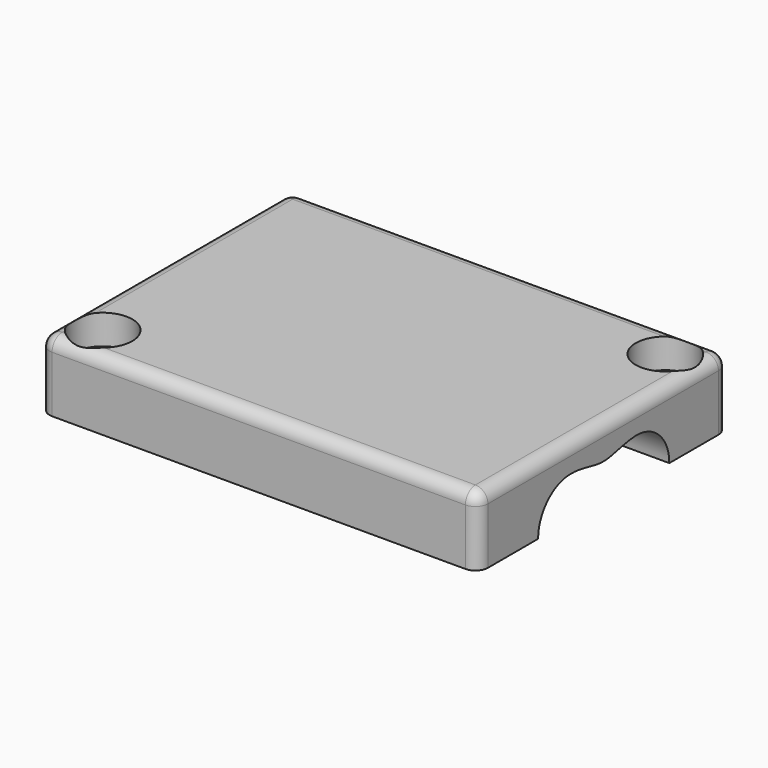
from build123d import *

# Parameters (mm, degrees)
F1_W          = 44.45
F1_H          = 31.75
F2_DEPTH      = 6.985
F4_DEPTH      = 44.45
F6_W          = 31.875
F6_H          = 1.75
F6_W_2        = 31.877
F7_DEPTH      = 2.5
F7_TAPER      = 7
F5_R          = 1.6
F8_DEPTH      = 25.4
F9_R          = 3
F9_R_2        = 1.6
F10_DEPTH     = 3
F11_T1_DEPTH  = 29.21
F11_T3_DEPTH  = 8.89
F11_T5_DEPTH  = 41.91
F11_S9_W      = 1.27
F11_S9_H      = 1.27
F11_T10_DEPTH = 1.27
F11_S15_W     = 1.27
F11_S15_H     = 1.27
F11_T16_DEPTH = 1.27
F11_S21_W     = 1.27
F11_S21_H     = 1.27
F11_T22_DEPTH = 1.27
F11_S27_W     = 1.27
F11_S27_H     = 1.27
F11_T28_DEPTH = 1.27


# Not quite as in the source:
# - a fillet or chamfer that OpenCascade refuses, or shapes differently, is made with other operations: its cross-section is extruded or revolved along the edge and cut away or added


with BuildPart() as f2:
    # F1 (on Top) → F2 (new body)
    with BuildSketch(Plane.XY):
        Rectangle(F1_W, F1_H)
    extrude(amount=F2_DEPTH)

    # F3 (on face) → F4 (cut, through all)
    with BuildSketch(Plane.YZ.offset(22.225)):
        with BuildLine():
            add(Edge.make_bspline(
                [(-4.125, 4.125), (-2.4255892558, 4.1137489608), (-0.0276085061, 2.971292738), (2.5249406681, 4.1137612248), (4.191, 4.191)],
                knots=[0, 0, 0, 0, 0.4977710734, 1, 1, 1, 1], degree=3))
            ThreePointArc((-4.125, 4.125), (-7.0418154724, 2.9168154724), (-8.25, 0))
            ThreePointArc((-8.25, 0), (-7.0418154724, -2.9168154724), (-4.125, -4.125))
            add(Edge.make_bspline(
                [(-4.125, -4.125), (-2.9335741419, -4.2006121948), (0.4172014685, -3.0581585459), (2.1438994445, -4.2006121948), (4.191, -4.191)],
                knots=[0, 0, 0, 0, 0.497799261, 1, 1, 1, 1], degree=3))
            ThreePointArc((4.191, -4.191), (7.15448452, -2.96348452), (8.382, 0))
            ThreePointArc((8.382, 0), (7.15448452, 2.96348452), (4.191, 4.191))
        make_face()
    extrude(amount=-F4_DEPTH, mode=Mode.SUBTRACT)

    # F6 (on Top) → F7 (cut)
    with BuildSketch(Plane.XY):
        with Locations((-4.4625, 13.175)):
            Rectangle(F6_W, F6_H)
        with Locations((4.4615, -13.175)):
            Rectangle(F6_W_2, F6_H)
    extrude(amount=F7_DEPTH, taper=F7_TAPER, mode=Mode.SUBTRACT)

    # F5 (on Top) → F8 (cut)
    with BuildSketch(Plane.XY):
        with Locations((-18.669, -12.319)):
            Circle(F5_R)
        with Locations((18.669, 12.319)):
            Circle(F5_R)
    extrude(amount=F8_DEPTH, mode=Mode.SUBTRACT)

    # F9 (on face) → F10 (cut)
    with BuildSketch(Plane.XY.offset(6.985)):
        with Locations((-18.669, -12.319)):
            Circle(F9_R)
        with Locations((-18.669, -12.319)):
            Circle(F9_R_2, mode=Mode.SUBTRACT)
        with Locations((18.669, 12.319)):
            Circle(F9_R)
        with Locations((18.669, 12.319)):
            Circle(F9_R_2, mode=Mode.SUBTRACT)
    extrude(amount=-F10_DEPTH, mode=Mode.SUBTRACT)

    # F11: fillet of radius 1.27 on 8 edges, made by hand

    # F11_s2 → F11_t1 (cut)
    with BuildSketch(Plane.XZ.offset(-14.605)):
        with BuildLine():
            ThreePointArc((-22.225, 5.715), (-21.8530256121, 6.6130256121), (-20.955, 6.985))
            Line((-20.955, 6.985), (-22.225, 6.985))
            Line((-22.225, 6.985), (-22.225, 5.715))
        make_face()
        with BuildLine():
            ThreePointArc((22.225, 5.715), (21.8530256121, 6.6130256121), (20.955, 6.985))
            Line((20.955, 6.985), (22.225, 6.985))
            Line((22.225, 6.985), (22.225, 5.715))
        make_face()
    extrude(amount=F11_T1_DEPTH, mode=Mode.SUBTRACT)

    # F11_s4 → F11_t3 (cut)
    with BuildSketch(Plane.XY.offset(-3.175)):
        with BuildLine():
            ThreePointArc((-22.225, -14.605), (-21.8530256121, -15.5030256121), (-20.955, -15.875))
            Line((-20.955, -15.875), (-22.225, -15.875))
            Line((-22.225, -15.875), (-22.225, -14.605))
        make_face()
        with BuildLine():
            ThreePointArc((22.225, -14.605), (21.8530256121, -15.5030256121), (20.955, -15.875))
            Line((20.955, -15.875), (22.225, -15.875))
            Line((22.225, -15.875), (22.225, -14.605))
        make_face()
        with BuildLine():
            ThreePointArc((20.955, 15.875), (21.8530256121, 15.5030256121), (22.225, 14.605))
            Line((22.225, 14.605), (22.225, 15.875))
            Line((22.225, 15.875), (20.955, 15.875))
        make_face()
        with BuildLine():
            ThreePointArc((-20.955, 15.875), (-21.8530256121, 15.5030256121), (-22.225, 14.605))
            Line((-22.225, 14.605), (-22.225, 15.875))
            Line((-22.225, 15.875), (-20.955, 15.875))
        make_face()
    extrude(amount=F11_T3_DEPTH, mode=Mode.SUBTRACT)

    # F11_s6 → F11_t5 (cut)
    with BuildSketch(Plane.YZ.offset(-20.955)):
        with BuildLine():
            ThreePointArc((-14.605, 6.985), (-15.5030256121, 6.6130256121), (-15.875, 5.715))
            Line((-15.875, 5.715), (-15.875, 6.985))
            Line((-15.875, 6.985), (-14.605, 6.985))
        make_face()
        with BuildLine():
            ThreePointArc((15.875, 5.715), (15.5030256121, 6.6130256121), (14.605, 6.985))
            Line((14.605, 6.985), (15.875, 6.985))
            Line((15.875, 6.985), (15.875, 5.715))
        make_face()
    extrude(amount=F11_T5_DEPTH, mode=Mode.SUBTRACT)


with BuildPart() as f11_tool8:
    # F11_s9 → F11_t10 (new body)
    with BuildSketch(Plane.XZ.offset(-14.605)):
        with Locations((-21.59, 6.35)):
            Rectangle(F11_S9_W, F11_S9_H)
    extrude(amount=-F11_T10_DEPTH)

    # F11_s11 → F11_t12 (revolve, cut)
    with BuildSketch(Plane(origin=(-20.955, 14.605, 5.715), x_dir=(0.7071067812, 0, -0.7071067812), z_dir=(0.7071067812, 0, 0.7071067812))):
        with BuildLine():
            ThreePointArc((0, -1.27), (1.27, 0), (0, 1.27))
            Line((0, 1.27), (0, -1.27))
        make_face()
    revolve(axis=Axis((-20.955, 14.605, 5.715), (0, 1, 0)), mode=Mode.SUBTRACT)


with BuildPart() as f2_1:
    add(f2.part)

    # F11_t7: cut F11_tool8
    add(f11_tool8.part, mode=Mode.SUBTRACT)


with BuildPart() as f11_tool14:
    # F11_s15 → F11_t16 (new body)
    with BuildSketch(Plane.XZ.offset(14.605)):
        with Locations((-21.59, 6.35)):
            Rectangle(F11_S15_W, F11_S15_H)
    extrude(amount=F11_T16_DEPTH)

    # F11_s17 → F11_t18 (revolve, cut)
    with BuildSketch(Plane(origin=(-20.955, -14.605, 5.715), x_dir=(0.7071067812, 0, -0.7071067812), z_dir=(-0.7071067812, 0, -0.7071067812))):
        with BuildLine():
            ThreePointArc((0, -1.27), (1.27, 0), (0, 1.27))
            Line((0, 1.27), (0, -1.27))
        make_face()
    revolve(axis=Axis((-20.955, -14.605, 5.715), (0, -1, 0)), mode=Mode.SUBTRACT)


with BuildPart() as f2_2:
    add(f2_1.part)

    # F11_t13: cut F11_tool14
    add(f11_tool14.part, mode=Mode.SUBTRACT)


with BuildPart() as f11_tool20:
    # F11_s21 → F11_t22 (new body)
    with BuildSketch(Plane.XZ.offset(14.605)):
        with Locations((21.59, 6.35)):
            Rectangle(F11_S21_W, F11_S21_H)
    extrude(amount=F11_T22_DEPTH)

    # F11_s23 → F11_t24 (revolve, cut)
    with BuildSketch(Plane(origin=(20.955, -14.605, 5.715), x_dir=(-0.7071067812, 0, -0.7071067812), z_dir=(-0.7071067812, 0, 0.7071067812))):
        with BuildLine():
            ThreePointArc((0, -1.27), (1.27, 0), (0, 1.27))
            Line((0, 1.27), (0, -1.27))
        make_face()
    revolve(axis=Axis((20.955, -14.605, 5.715), (0, -1, 0)), mode=Mode.SUBTRACT)


with BuildPart() as f2_3:
    add(f2_2.part)

    # F11_t19: cut F11_tool20
    add(f11_tool20.part, mode=Mode.SUBTRACT)


with BuildPart() as f11_tool26:
    # F11_s27 → F11_t28 (new body)
    with BuildSketch(Plane.XZ.offset(-14.605)):
        with Locations((21.59, 6.35)):
            Rectangle(F11_S27_W, F11_S27_H)
    extrude(amount=-F11_T28_DEPTH)

    # F11_s29 → F11_t30 (revolve, cut)
    with BuildSketch(Plane(origin=(20.955, 14.605, 5.715), x_dir=(-0.7071067812, 0, -0.7071067812), z_dir=(0.7071067812, 0, -0.7071067812))):
        with BuildLine():
            ThreePointArc((0, -1.27), (1.27, 0), (0, 1.27))
            Line((0, 1.27), (0, -1.27))
        make_face()
    revolve(axis=Axis((20.955, 14.605, 5.715), (0, 1, 0)), mode=Mode.SUBTRACT)


with BuildPart() as f2_4:
    add(f2_3.part)

    # F11_t25: cut F11_tool26
    add(f11_tool26.part, mode=Mode.SUBTRACT)


solid = f2_4.part
